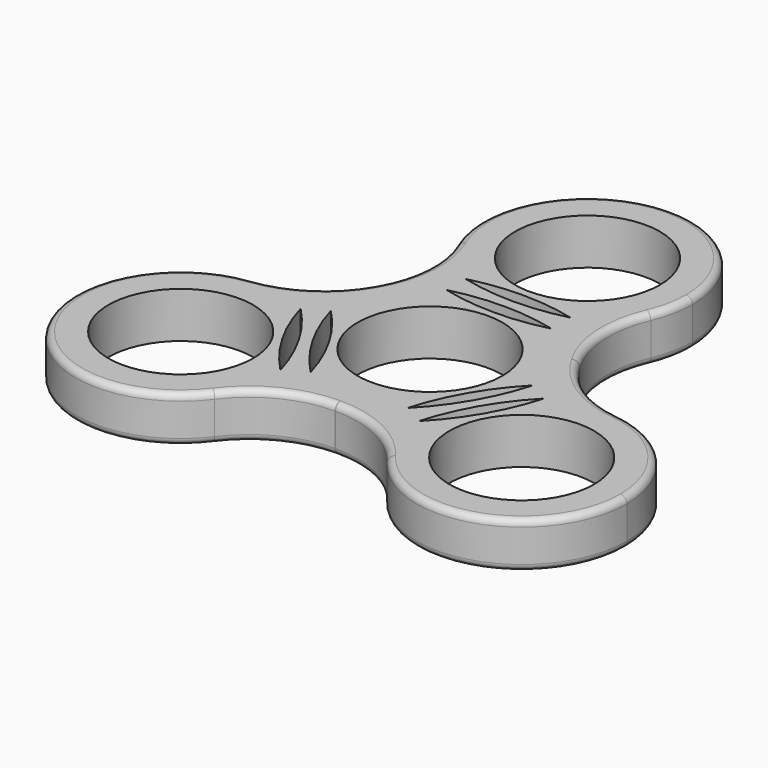
from build123d import *

# Parameters (mm, degrees)
F0_R     = 11.025
F1_DEPTH = 7
F2_R     = 1
F4_DEPTH = 25


with BuildPart() as f1:
    # F0 (on Top) → F1 (new body)
    with BuildSketch(Plane.XY):
        with BuildLine():
            ThreePointArc((14.7181475974, 23.6614862702), (15.6948867509, 26.7640836111), (16.025, 30))
            ThreePointArc((16.025, 30), (-3.2359163889, 45.6948867509), (-14.7181475974, 23.6614862702))
            ThreePointArc((-14.7181475974, 23.6614862702), (-11.9828737003, 19.359917158), (-8.0350731173, 16.135))
            ThreePointArc((-8.0350731173, 16.135), (0, 18.025), (8.0350731173, 16.135))
            ThreePointArc((8.0350731173, 16.135), (11.9828737003, 19.359917158), (14.7181475974, 23.6614862702))
        make_face()
        with Locations((0, 30)):
            Circle(F0_R, mode=Mode.SUBTRACT)
        with BuildLine():
            ThreePointArc((-8.0350731173, 16.135), (-11.9828737003, 19.359917158), (-14.7181475974, 23.6614862702))
            ThreePointArc((-14.7181475974, 23.6614862702), (-13.4190857224, 16.250871043), (-15.58998593, 9.0472627741))
            ThreePointArc((-15.58998593, 9.0472627741), (-12.3326744258, 13.1455607149), (-8.0350731173, 16.135))
        make_face()
        with BuildLine():
            ThreePointArc((15.58998593, 9.0472627741), (13.4190857224, 16.250871043), (14.7181475974, 23.6614862702))
            ThreePointArc((14.7181475974, 23.6614862702), (11.9828737003, 19.359917158), (8.0350731173, 16.135))
            ThreePointArc((8.0350731173, 16.135), (12.3326744258, 13.1455607149), (15.58998593, 9.0472627741))
        make_face()
        with BuildLine():
            ThreePointArc((8.0350731173, 16.135), (0, 13.975), (-8.0350731173, 16.135))
            ThreePointArc((-8.0350731173, 16.135), (-12.3326744258, 13.1455607149), (-15.58998593, 9.0472627741))
            ThreePointArc((-15.58998593, 9.0472627741), (-15.6101079032, 9.0125), (-15.6301523621, 8.9776924729))
            ThreePointArc((-15.6301523621, 8.9776924729), (-17.5507267389, 4.1076289919), (-17.9908564487, -1.1089225592))
            ThreePointArc((-17.9908564487, -1.1089225592), (-12.1092289741, -6.9762107854), (-9.9557621135, -15))
            ThreePointArc((-9.9557621135, -15), (-9.955767418, -15.0130387247), (-9.9557833314, -15.0260774408))
            ThreePointArc((-9.9557833314, -15.0260774408), (-5.2180523132, -17.2531897067), (-0.0401664321, -18.024955247))
            ThreePointArc((-0.0401664321, -18.024955247), (0, -18.025), (0.0401664321, -18.024955247))
            ThreePointArc((0.0401664321, -18.024955247), (5.2180523132, -17.2531897067), (9.9557833314, -15.0260774408))
            ThreePointArc((9.9557833314, -15.0260774408), (12.1027050179, -6.9875), (17.9908564487, -1.1089225592))
            ThreePointArc((17.9908564487, -1.1089225592), (18.0164620901, -0.554724036), (18.025, 0))
            ThreePointArc((18.025, 0), (17.4160001339, 4.6458114831), (15.6301523621, 8.9776924729))
            ThreePointArc((15.6301523621, 8.9776924729), (15.6101079032, 9.0125), (15.58998593, 9.0472627741))
            ThreePointArc((15.58998593, 9.0472627741), (12.3326744258, 13.1455607149), (8.0350731173, 16.135))
        make_face()
        Circle(F0_R, mode=Mode.SUBTRACT)
        with BuildLine():
            ThreePointArc((-17.9908564487, -1.1089225592), (-17.5507267389, 4.1076289919), (-15.6301523621, 8.9776924729))
            ThreePointArc((-15.6301523621, 8.9776924729), (-20.783210018, 3.4958336097), (-27.850522, 0.9155465808))
            ThreePointArc((-27.850522, 0.9155465808), (-22.7576169242, 0.6975144557), (-17.9908564487, -1.1089225592))
        make_face()
        with BuildLine():
            ThreePointArc((27.850522, 0.9155465808), (20.783210018, 3.4958336097), (15.6301523621, 8.9776924729))
            ThreePointArc((15.6301523621, 8.9776924729), (17.4160001339, 4.6458114831), (18.025, 0))
            ThreePointArc((18.025, 0), (18.0164620901, -0.554724036), (17.9908564487, -1.1089225592))
            ThreePointArc((17.9908564487, -1.1089225592), (22.7576169242, 0.6975144557), (27.850522, 0.9155465808))
        make_face()
        with BuildLine():
            ThreePointArc((-9.9557833314, -15.0260774408), (-15.6101079032, -9.0125), (-17.9908564487, -1.1089225592))
            ThreePointArc((-17.9908564487, -1.1089225592), (-22.7576169242, 0.6975144557), (-27.850522, 0.9155465808))
            ThreePointArc((-27.850522, 0.9155465808), (-39.8588192092, -23.0125), (-13.1323744027, -24.5770328511))
            ThreePointArc((-13.1323744027, -24.5770328511), (-10.7747432239, -20.0574316138), (-9.9557833314, -15.0260774408))
        make_face()
        with Locations((-25.9807621135, -15)):
            Circle(F0_R, mode=Mode.SUBTRACT)
        with BuildLine():
            ThreePointArc((42.0057621135, -15), (37.9549745549, -4.3501708272), (27.850522, 0.9155465808))
            ThreePointArc((27.850522, 0.9155465808), (22.7576169242, 0.6975144557), (17.9908564487, -1.1089225592))
            ThreePointArc((17.9908564487, -1.1089225592), (15.6101079032, -9.0125), (9.9557833314, -15.0260774408))
            ThreePointArc((9.9557833314, -15.0260774408), (10.7747432239, -20.0574316138), (13.1323744027, -24.5770328511))
            ThreePointArc((13.1323744027, -24.5770328511), (31.0258196917, -30.2101288303), (42.0057621135, -15))
        make_face()
        with Locations((25.9807621135, -15)):
            Circle(F0_R, mode=Mode.SUBTRACT)
        with BuildLine():
            ThreePointArc((-0.0401664321, -18.024955247), (-5.2180523132, -17.2531897067), (-9.9557833314, -15.0260774408))
            ThreePointArc((-9.9557833314, -15.0260774408), (-10.7747432239, -20.0574316138), (-13.1323744027, -24.5770328511))
            ThreePointArc((-13.1323744027, -24.5770328511), (-7.3641242956, -19.7467046526), (-0.0401664321, -18.024955247))
        make_face()
        with BuildLine():
            ThreePointArc((13.1323744027, -24.5770328511), (10.7747432239, -20.0574316138), (9.9557833314, -15.0260774408))
            ThreePointArc((9.9557833314, -15.0260774408), (5.2180523132, -17.2531897067), (0.0401664321, -18.024955247))
            ThreePointArc((0.0401664321, -18.024955247), (7.3641242956, -19.7467046526), (13.1323744027, -24.5770328511))
        make_face()
        with BuildLine():
            ThreePointArc((-9.9557621135, -15), (-12.1092289741, -6.9762107854), (-17.9908564487, -1.1089225592))
            ThreePointArc((-17.9908564487, -1.1089225592), (-15.6101079032, -9.0125), (-9.9557833314, -15.0260774408))
            ThreePointArc((-9.9557833314, -15.0260774408), (-9.955767418, -15.0130387247), (-9.9557621135, -15))
        make_face()
        with BuildLine():
            ThreePointArc((8.0350731173, 16.135), (0, 18.025), (-8.0350731173, 16.135))
            ThreePointArc((-8.0350731173, 16.135), (0, 13.975), (8.0350731173, 16.135))
        make_face()
        with BuildLine():
            ThreePointArc((9.9557833314, -15.0260774408), (15.6101079032, -9.0125), (17.9908564487, -1.1089225592))
            ThreePointArc((17.9908564487, -1.1089225592), (12.1027050179, -6.9875), (9.9557833314, -15.0260774408))
        make_face()
    extrude(amount=F1_DEPTH)

    # F2
    f2_edges = [f1.edges().sort_by_distance(p)[0] for p in [
        (14.718148, 23.661486, 3.5),
        (-14.718148, 23.661486, 3.5),
        (0, 46.025, 0),
        (0, 46.025, 7),
        (-15.589986, 9.047263, 3.5),
        (-13.419086, 16.250871, 0),
        (-13.419086, 16.250871, 7),
        (-15.630152, 8.977692, 3.5),
        (-27.850522, 0.915547, 3.5),
        (-20.78321, 3.495834, 0),
        (-20.78321, 3.495834, 7),
        (-13.132374, -24.577033, 3.5),
        (-39.858819, -23.0125, 0),
        (-39.858819, -23.0125, 7),
        (0.040166, -18.024955, 3.5),
        (13.132374, -24.577033, 3.5),
        (7.364124, -19.746705, 0),
        (7.364124, -19.746705, 7),
    ]]
    fillet(f2_edges, radius=F2_R)

    # F3 (on face) → F4 (cut)
    with BuildSketch(Plane.XY.offset(7)):
        with BuildLine():
            ThreePointArc((-8, 16.7844323657), (0, 15.7868354251), (8, 16.7844323657))
            ThreePointArc((8, 16.7844323657), (0, 17.7820293063), (-8, 16.7844323657))
        make_face()
        with BuildLine():
            ThreePointArc((-8, 13.1454704053), (0, 12.1478734647), (8, 13.1454704053))
            ThreePointArc((8, 13.1454704053), (0, 14.1430673459), (-8, 13.1454704053))
        make_face()
        with BuildLine():
            ThreePointArc((-15.3843113157, 0.3554680276), (-12.248255609, -7.0715336729), (-7.3843113157, -13.5009384329))
            ThreePointArc((-7.3843113157, -13.5009384329), (-10.5203670224, -6.0739367324), (-15.3843113157, 0.3554680276))
        make_face()
        with BuildLine():
            ThreePointArc((-18.5357448168, -1.4640129526), (-15.3996891101, -8.8910146531), (-10.5357448168, -15.3204194131))
            ThreePointArc((-10.5357448168, -15.3204194131), (-13.6718005235, -7.8934177126), (-18.5357448168, -1.4640129526))
        make_face()
        with BuildLine():
            ThreePointArc((7.3843113157, -13.5009384329), (12.248255609, -7.0715336729), (15.3843113157, 0.3554680276))
            ThreePointArc((15.3843113157, 0.3554680276), (10.5203670224, -6.0739367324), (7.3843113157, -13.5009384329))
        make_face()
        with BuildLine():
            ThreePointArc((10.5357448168, -15.3204194131), (15.3996891101, -8.8910146531), (18.5357448168, -1.4640129526))
            ThreePointArc((18.5357448168, -1.4640129526), (13.6718005235, -7.8934177126), (10.5357448168, -15.3204194131))
        make_face()
    extrude(amount=-F4_DEPTH, mode=Mode.SUBTRACT)


solid = f1.part
